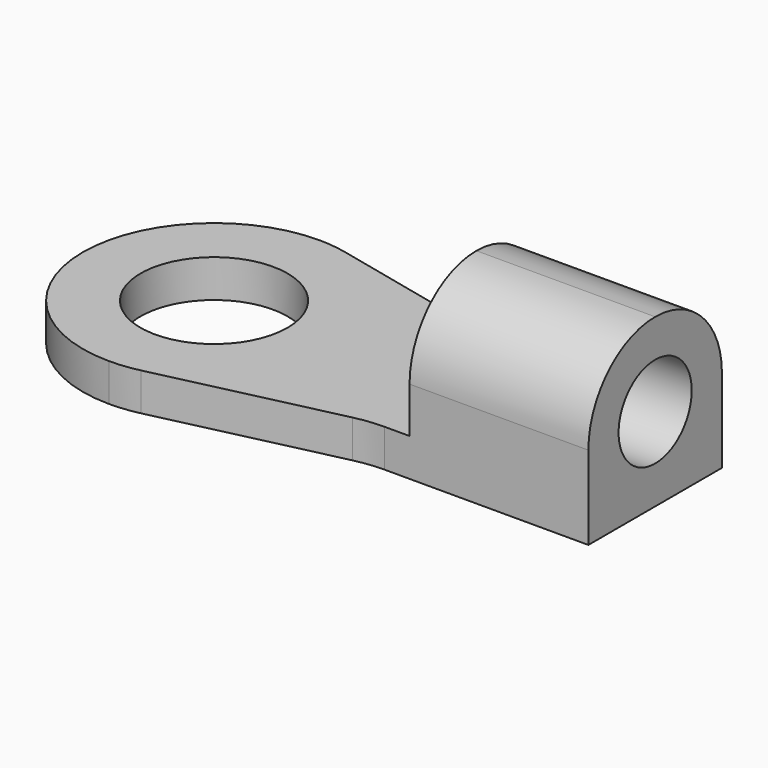
from build123d import *

# Parameters (mm, degrees)
F0_R     = 1.85
F1_DEPTH = 0.95
F2_W     = 4.5
F2_H     = 4.2
F3_DEPTH = 3.25
F4_R     = 2.09999
F5_R     = 1.15
F6_DEPTH = 25


# Not quite as in the source:
# - a fillet or chamfer is up to 0.001 mm smaller than in the source, because OpenCascade refuses the exact size


with BuildPart() as f1:
    # F0 (on Top) → F1 (new body)
    with BuildSketch(Plane.XY):
        with BuildLine():
            Line((9.2740088212, 1.2), (14.4, 1.2))
            Line((14.4, 1.2), (14.4, 5.4))
            Line((14.4, 5.4), (9.2740088212, 5.4))
            ThreePointArc((9.2740088212, 5.4), (8.9023791849, 5.4209923127), (8.5354776489, 5.4837021737))
            Line((8.5354776489, 5.4837021737), (4.0385311723, 6.5162978263))
            ThreePointArc((4.0385311723, 6.5162978263), (3.6716296363, 6.5790076873), (3.3, 6.6))
            ThreePointArc((3.3, 6.6), (0.9665476221, 5.6334523779), (0, 3.3))
            ThreePointArc((0, 3.3), (0.9665476221, 0.9665476221), (3.3, 0))
            ThreePointArc((3.3, 0), (3.6716296363, 0.0209923127), (4.0385311723, 0.0837021737))
            Line((4.0385311723, 0.0837021737), (8.5354776489, 1.1162978263))
            ThreePointArc((8.5354776489, 1.1162978263), (8.9023791849, 1.1790076873), (9.2740088212, 1.2))
        make_face()
        with Locations((3.3, 3.3)):
            Circle(F0_R, mode=Mode.SUBTRACT)
    extrude(amount=F1_DEPTH)

    # F2 (on face) → F3 (join)
    with BuildSketch(Plane.XY.offset(0.95)):
        with Locations((12.15, 3.3)):
            Rectangle(F2_W, F2_H)
    extrude(amount=F3_DEPTH)

    # F4 (radius 2.1 in the source; OpenCascade refuses exactly that, so slightly less here)
    f4_edges = [f1.edges().sort_by_distance(p)[0] for p in [
        (12.15, 5.4, 4.2),
        (12.15, 1.2, 4.2),
    ]]
    fillet(f4_edges, radius=F4_R)

    # F5 (on face) → F6 (cut)
    with BuildSketch(Plane.YZ.offset(14.4)):
        with Locations((3.3, 2.1)):
            Circle(F5_R)
    extrude(amount=-F6_DEPTH, mode=Mode.SUBTRACT)


solid = f1.part
